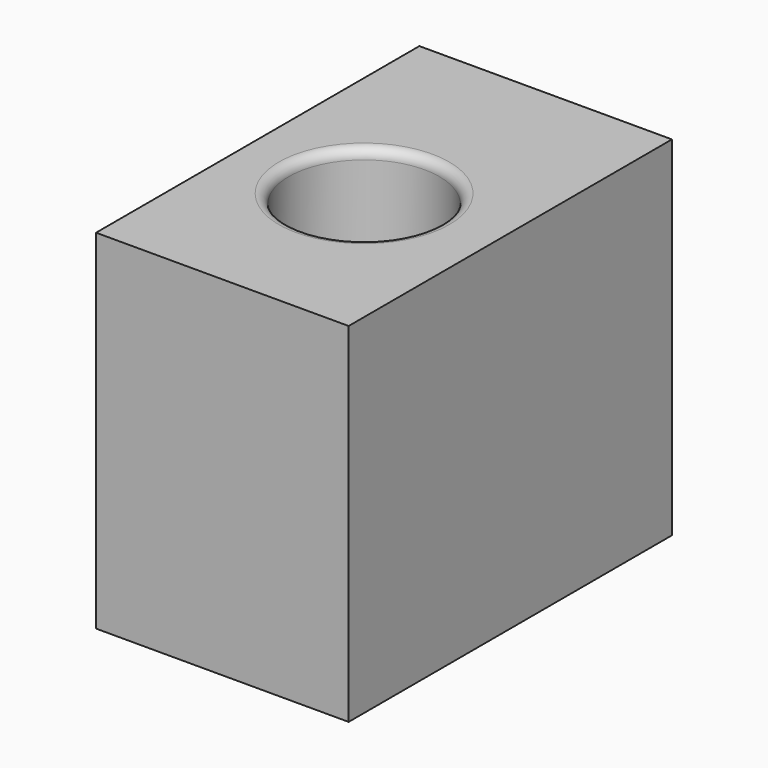
from build123d import *

# Parameters (mm, degrees)
F0_W     = 25
F0_H     = 40
F1_DEPTH = 25
F2_W     = 25
F2_H     = 40
F2_R     = 7.4574120062
F3_DEPTH = 9.5
F5_R     = 0.9656854249


# Not quite as in the source:
# - the program builds the solid bodies; features that only make, move or delete a surface that nothing else refers to are left out


with BuildPart() as f1:
    # F0 (on Top) → F1 (new body)
    with BuildSketch(Plane.XY):
        with Locations((0.5926040933, 1.8275822699)):
            Rectangle(F0_W, F0_H)
    extrude(amount=F1_DEPTH)

    # F2 (on face) → F3 (join)
    with BuildSketch(Plane.XY.offset(25)):
        with Locations((0.5926040933, 1.8275822699)):
            Rectangle(F2_W, F2_H)
        with Locations((0.1519261859, -0.08621795)):
            Circle(F2_R, mode=Mode.SUBTRACT)
    extrude(amount=F3_DEPTH)

    # F5
    f5_edges = [f1.edges().sort_by_distance(p)[0] for p in [
        (-7.305486, -0.086218, 34.5),
    ]]
    fillet(f5_edges, radius=F5_R)


solid = f1.part
